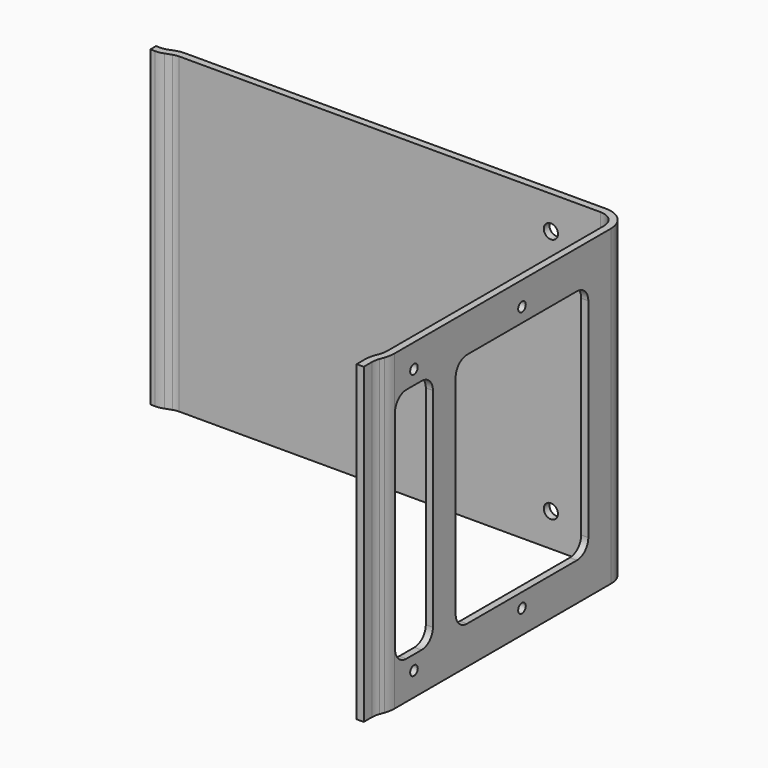
from build123d import *

# Parameters (mm, degrees)
F1_DEPTH  = 66
F2_R      = 1.5
F3_DEPTH  = 25
F4_R      = 1
F5_DEPTH  = 25
F6_R      = 5
F7_R      = 6.5
F8_W      = 11.5
F8_H      = 48
F9_DEPTH  = 100
F11_DEPTH = 66


# Not quite as in the source:
# - a feature names something its author has since deleted; it is built from what else it names


with BuildPart() as f1:
    # F0 (on Top) → F1 (new body)
    with BuildSketch(Plane.XY):
        with BuildLine():
            Line((54.5, 33), (54.5, -24.9880321095))
            Line((54.5, -24.9880321095), (53.5, -27.7355095289))
            Line((53.5, -27.7355095289), (53.5, -31))
            Line((53.5, -31), (55, -31))
            Line((55, -31), (55, -28))
            Line((55, -28), (56, -25.2525225805))
            Line((56, -25.2525225805), (56, 33))
            ThreePointArc((56, 33), (54.5355339059, 36.5355339059), (51, 38))
            Line((51, 38), (-42.5, 38))
            ThreePointArc((-42.5, 38), (-46.0355339059, 36.5355339059), (-47.5, 33))
            Line((-47.5, 33), (-47.5, 0))
            Line((-47.5, 0), (-46.000000001, 0))
            Line((-46.000000001, 0), (-46.000000001, 33))
            ThreePointArc((-46.000000001, 33), (-44.9748737349, 35.4748737349), (-42.5, 36.500000001))
            Line((-42.5, 36.5), (51, 36.5))
            ThreePointArc((51, 36.5), (53.4748737342, 35.4748737342), (54.5, 33))
        make_face()
    extrude(amount=F1_DEPTH)

    # F2 (on face) → F3 (cut)
    with BuildSketch(Plane(origin=(0, 38, 0), x_dir=(-1, 0, 0), z_dir=(0, 1, 0))):
        with Locations((-40.5, 59)):
            Circle(F2_R)
        with Locations((-40.5, 7)):
            Circle(F2_R)
    extrude(amount=-F3_DEPTH, mode=Mode.SUBTRACT)

    # F4 (on face) → F5 (cut)
    with BuildSketch(Plane.YZ.offset(56)):
        with BuildLine():
            Line((-17, 58), (-21, 58))
            ThreePointArc((-21, 58), (-23.1213203436, 57.1213203436), (-24, 55))
            Line((-24, 55), (-24, 11))
            ThreePointArc((-24, 11), (-23.1213203436, 8.8786796564), (-21, 8))
            Line((-21, 8), (-17, 8))
            ThreePointArc((-17, 8), (-14.8786796564, 8.8786796564), (-14, 11))
            Line((-14, 11), (-14, 55))
            ThreePointArc((-14, 55), (-14.8786796564, 57.1213203436), (-17, 58))
        make_face()
        with BuildLine():
            Line((24, 58), (-5, 58))
            ThreePointArc((-5, 58), (-7.1213203436, 57.1213203436), (-8, 55))
            Line((-8, 55), (-8, 11))
            ThreePointArc((-8, 11), (-7.1213203436, 8.8786796564), (-5, 8))
            Line((-5, 8), (24, 8))
            ThreePointArc((24, 8), (26.1213203436, 8.8786796564), (27, 11))
            Line((27, 11), (27, 55))
            ThreePointArc((27, 55), (26.1213203436, 57.1213203436), (24, 58))
        make_face()
        with Locations((-19, 61)):
            Circle(F4_R)
        with Locations((9.5, 61)):
            Circle(F4_R)
        with Locations((9.5, 5)):
            Circle(F4_R)
        with Locations((-19, 5)):
            Circle(F4_R)
    extrude(amount=-F5_DEPTH, mode=Mode.SUBTRACT)

    # F6
    f6_edges = [f1.edges().sort_by_distance(p)[0] for p in [
        (55, -28, 33),
        (54.5, -24.988032, 33),
    ]]
    fillet(f6_edges, radius=F6_R)

    # F7
    f7_edges = [f1.edges().sort_by_distance(p)[0] for p in [
        (56, -25.252523, 33),
        (53.5, -27.73551, 33),
    ]]
    fillet(f7_edges, radius=F7_R)

    # F8 (on Top) → F9 (cut)
    with BuildSketch(Plane.XY):
        with Locations((-43.75, 19)):
            Rectangle(F8_W, F8_H)
    extrude(amount=F9_DEPTH, mode=Mode.SUBTRACT)

    # F10 (on Top) → F11 (join)
    with BuildSketch(Plane.XY):
        with BuildLine():
            Line((-43.2462567555, 37), (-43.2462567555, 35.5))
            Line((-43.2462567555, 35.5), (-42.2462567555, 35.5))
            ThreePointArc((-42.2462567555, 35.5), (-41.3780158671, 35.5759612349), (-40.5361560388, 35.8015368961))
            Line((-40.5361560388, 35.8015368961), (-39.1970705016, 36.2889241728))
            ThreePointArc((-39.1970705016, 36.2889241728), (-38.6077686218, 36.4468271355), (-38, 36.5))
            Line((-38, 36.5), (-38, 38))
            ThreePointArc((-38, 38), (-38.8682408883, 37.9240387651), (-39.7101007166, 37.6984631039))
            Line((-39.7101007166, 37.6984631039), (-41.0491862538, 37.2110758272))
            ThreePointArc((-41.0491862538, 37.2110758272), (-41.6384881336, 37.0531728645), (-42.2462567555, 37))
            Line((-42.2462567555, 37), (-43.2462567555, 37))
        make_face()
    extrude(amount=F11_DEPTH)


solid = f1.part
